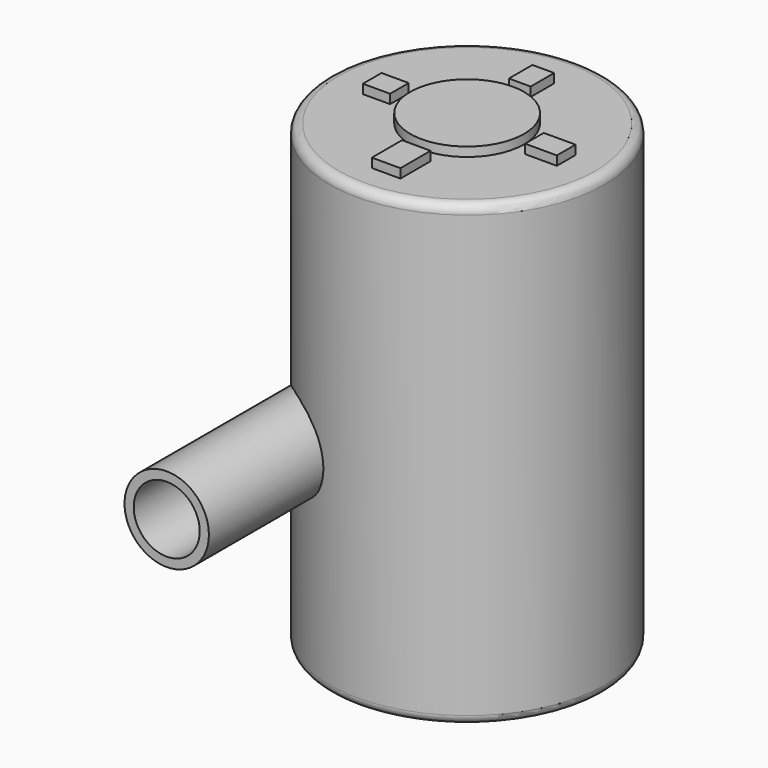
from build123d import *

# Parameters (mm, degrees)
F0_R      = 76.2
F1_DEPTH  = 254
F2_R      = 31.5064742485
F3_DEPTH  = 5.08
F5_R      = 5.08
F6_R      = 5.08
F7_W      = 15.0262638927
F7_H      = 12.87966175
F8_DEPTH  = 5.08
F9_W      = 12.0340203866
F9_H      = 16.2621960044
F10_DEPTH = 5.08
F11_W     = 17.5631716847
F11_H     = 12.9121849313
F12_DEPTH = 5.08
F13_W     = 15.818908345
F13_H     = 20.8626762033
F14_DEPTH = 5.08
F15_R     = 23.3473489608
F16_DEPTH = 152.4
F18_T     = -5.08


# Not quite as in the source:
# - a feature of the source that left no trace in its solid (it failed there, or was rolled back) is left out


with BuildPart() as f1:
    # F0 (on Top) → F1 (new body)
    with BuildSketch(Plane.XY):
        Circle(F0_R)
    extrude(amount=F1_DEPTH)

    # F5
    f5_edges = [f1.edges().sort_by_distance(p)[0] for p in [
        (-76.2, 0, 254),
    ]]
    fillet(f5_edges, radius=F5_R)

    # F6
    f6_edges = [f1.edges().sort_by_distance(p)[0] for p in [
        (-76.2, 0, 0),
    ]]
    fillet(f6_edges, radius=F6_R)


with BuildPart() as f3:
    # F2 (on face) → F3 (new body)
    with BuildSketch(Plane.XY.offset(254)):
        Circle(F2_R)
    extrude(amount=F3_DEPTH)


with BuildPart() as f8:
    # F7 (on face) → F8 (new body)
    with BuildSketch(Plane.XY.offset(254)):
        with Locations((-44.7210334241, -0.3577677999)):
            Rectangle(F7_W, F7_H)
    extrude(amount=F8_DEPTH)


with BuildPart() as f10:
    # F9 (on face) → F10 (new body)
    with BuildSketch(Plane.XY.offset(254)):
        with Locations((0, 44.558417052)):
            Rectangle(F9_W, F9_H)
    extrude(amount=F10_DEPTH)


with BuildPart() as f12:
    # F11 (on face) → F12 (new body)
    with BuildSketch(Plane.XY.offset(254)):
        with Locations((46.3472604752, -0.3740293905)):
            Rectangle(F11_W, F11_H)
    extrude(amount=F12_DEPTH)


with BuildPart() as f14:
    # F13 (on face) → F14 (new body)
    with BuildSketch(Plane.XY.offset(254)):
        with Locations((1.8924439792, -47.9520522058)):
            Rectangle(F13_W, F13_H)
    extrude(amount=F14_DEPTH)


with BuildPart() as f16:
    # F15 (on Front) → F16 (new body)
    with BuildSketch(Plane.XZ):
        with Locations((-44.3437509239, -31.4783900976)):
            Circle(F15_R)
    extrude(amount=F16_DEPTH)


with BuildPart() as f16_1:
    # F17: moved
    add(f16.part.moved(Location((0, 0, 140.14199))))

    # F18
    f18_openings = [f16_1.faces().sort_by_distance(p)[0] for p in [
        (-44.343751, -152.4, 108.6636),
    ]]
    offset(amount=F18_T, openings=f18_openings)


solid = Compound([f1.part, f3.part, f8.part, f10.part, f12.part, f14.part, f16_1.part])
